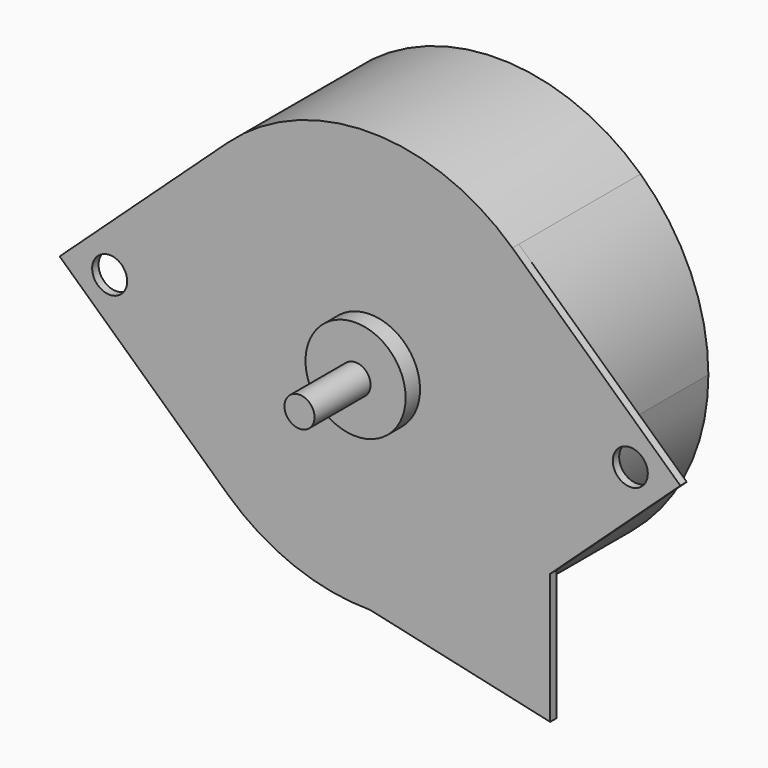
from build123d import *

# Parameters (mm, degrees)
F0_R     = 1.5
F1_DEPTH = 8.8
F0_R_2   = 5
F2_DEPTH = 1.8
F3_DEPTH = 16
F0_R_3   = 1.75
F4_DEPTH = 0.8


with BuildPart() as f1:
    # F0 (on Front) → F1 (new body)
    with BuildSketch(Plane.XZ):
        Circle(F0_R)
    extrude(amount=F1_DEPTH)


with BuildPart() as f2:
    # F0 (on Front) → F2 (new body)
    with BuildSketch(Plane.XZ):
        Circle(F0_R_2)
        Circle(F0_R, mode=Mode.SUBTRACT)
    extrude(amount=F2_DEPTH)

    # F0 (on Front) → F3 (join)
    with BuildSketch(Plane.XZ):
        with BuildLine():
            ThreePointArc((0, -21), (14.8492424049, -14.8492424049), (21, 0))
            ThreePointArc((21, 0), (19.2320297354, 8.4338029535), (14.2258064516, 15.4475380175))
            ThreePointArc((14.2258064516, 15.4475380175), (0, 21), (-14.2258064516, 15.4475380175))
            ThreePointArc((-14.2258064516, 15.4475380175), (-21, 0), (-14.2258064516, -15.4475380175))
            ThreePointArc((-14.2258064516, -15.4475380175), (-7.6354993823, -19.5626979015), (0, -21))
        make_face()
        Circle(F0_R_2, mode=Mode.SUBTRACT)
        Circle(F0_R_2)
        Circle(F0_R, mode=Mode.SUBTRACT)
    extrude(amount=-F3_DEPTH)

    # F0 (on Front) → F4 (join)
    with BuildSketch(Plane.XZ):
        with BuildLine():
            ThreePointArc((-14.2258064516, -15.4475380175), (-21, 0), (-14.2258064516, 15.4475380175))
            Line((-14.2258064516, 15.4475380175), (-31, 0))
            Line((-31, 0), (-14.2258064516, -15.4475380175))
        make_face()
        with Locations((-26, 0)):
            Circle(F0_R_3, mode=Mode.SUBTRACT)
        with BuildLine():
            ThreePointArc((14.2258064516, 15.4475380175), (19.2320297354, 8.4338029535), (21, 0))
            ThreePointArc((21, 0), (14.8492424049, -14.8492424049), (0, -21))
            Line((0, -21), (18, -25))
            Line((18, -25), (18, -11.9718419635))
            Line((18, -11.9718419635), (31, 0))
            Line((31, 0), (14.2258064516, 15.4475380175))
        make_face()
        with Locations((26, 0)):
            Circle(F0_R_3, mode=Mode.SUBTRACT)
        with BuildLine():
            ThreePointArc((0, -21), (14.8492424049, -14.8492424049), (21, 0))
            ThreePointArc((21, 0), (19.2320297354, 8.4338029535), (14.2258064516, 15.4475380175))
            ThreePointArc((14.2258064516, 15.4475380175), (0, 21), (-14.2258064516, 15.4475380175))
            ThreePointArc((-14.2258064516, 15.4475380175), (-21, 0), (-14.2258064516, -15.4475380175))
            ThreePointArc((-14.2258064516, -15.4475380175), (-7.6354993823, -19.5626979015), (0, -21))
        make_face()
        Circle(F0_R_2, mode=Mode.SUBTRACT)
    extrude(amount=-F4_DEPTH)


solid = Compound([f1.part, f2.part])
